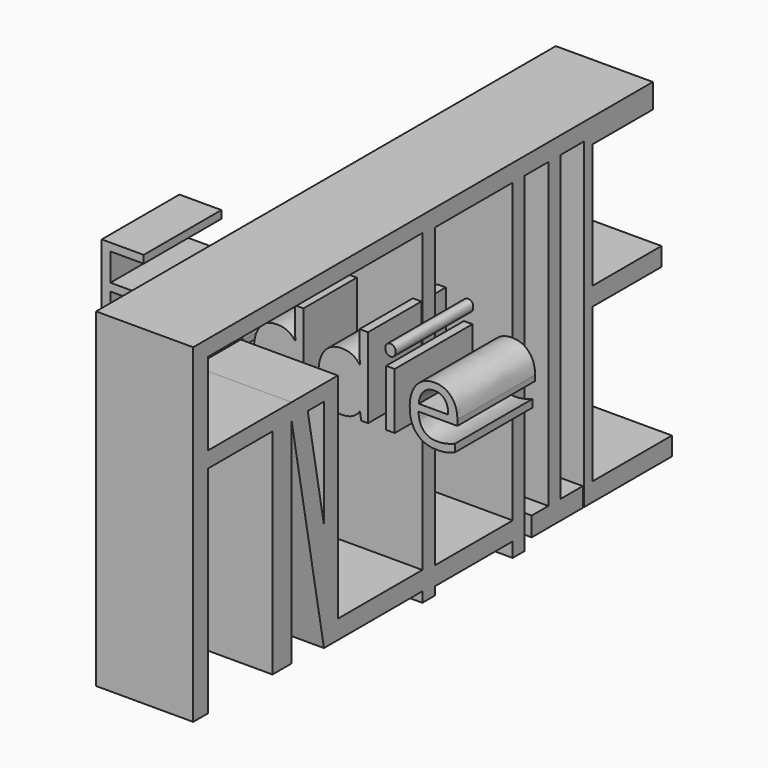
from build123d import *

# Parameters (mm, degrees)
F0_TEXT_SIZE = 27.5686564338
F1_DEPTH     = 25.4
F2_W         = 21.0011973977
F2_H         = 4.1624009609
F2_W_2       = 6.2435939908
F2_H_2       = 56.003193371
F2_W_3       = 27.6231979951
F2_H_3       = 4.9192011356
F2_W_4       = 4.0206052363
F2_H_4       = 79.2058780789
F2_H_5       = 5.025755614
F2_W_5       = 5.4278131574
F2_W_6       = 7.2370879352
F2_W_7       = 22.515386343
F2_H_6       = 4.8247235827
F2_W_8       = 25.9328857064
F2_H_7       = 4.8247240484
F3_DEPTH     = 25.4


# Not quite as in the source:
# - Text() gives the source's letters only with a copy of the font that has no kerning and outlines rounded to 1/6400 em; it was checked with that copy


with BuildPart() as f1:
    # F0 (on Front) → F1 (new body)
    with BuildSketch(Plane.XZ):
        with BuildLine():
            add(Edge.make_bspline(
                [(15.5439399558, 3.0433212141), (16.5799183734, 1.6024281552), (18.58726117, 1.6024281552)],
                knots=[0, 0, 0, 1, 1, 1], degree=2))
            add(Edge.make_bspline(
                [(18.58726117, 1.6024281552), (20.8745981335, 1.6024281552), (21.9041151472, 2.8473252973)],
                knots=[0, 0, 0, 1, 1, 1], degree=2))
            add(Edge.make_bspline(
                [(21.9041151472, 2.8473252973), (22.9336321609, 4.0922224394), (22.9336321609, 6.866318493)],
                knots=[0, 0, 0, 1, 1, 1], degree=2))
            Line((22.9336321609, 6.866318493), (22.9336321609, 7.3358471729))
            add(Edge.make_bspline(
                [(22.9336321609, 7.3358471729), (22.9336321609, 10.4717818423), (21.8911923395, 11.8114462409)],
                knots=[0, 0, 0, 1, 1, 1], degree=2))
            add(Edge.make_bspline(
                [(21.8911923395, 11.8114462409), (20.8487525181, 13.1511106394), (18.5614155546, 13.1511106394)],
                knots=[0, 0, 0, 1, 1, 1], degree=2))
            add(Edge.make_bspline(
                [(18.5614155546, 13.1511106394), (16.5928411811, 13.1511106394), (15.5504013597, 11.6240655292)],
                knots=[0, 0, 0, 1, 1, 1], degree=2))
            add(Edge.make_bspline(
                [(15.5504013597, 11.6240655292), (14.5079615383, 10.0970204189), (14.5079615383, 7.3100015575)],
                knots=[0, 0, 0, 1, 1, 1], degree=2))
            add(Edge.make_bspline(
                [(14.5079615383, 7.3100015575), (14.5079615383, 4.4842142731), (15.5439399558, 3.0433212141)],
                knots=[0, 0, 0, 1, 1, 1], degree=2))
        make_face()
        with BuildLine():
            add(Edge.make_bspline(
                [(-1.350477315, 3.0433212141), (-0.3144988974, 1.6024281552), (1.6928438991, 1.6024281552)],
                knots=[0, 0, 0, 1, 1, 1], degree=2))
            add(Edge.make_bspline(
                [(1.6928438991, 1.6024281552), (3.9801808626, 1.6024281552), (5.0096978763, 2.8473252973)],
                knots=[0, 0, 0, 1, 1, 1], degree=2))
            add(Edge.make_bspline(
                [(5.0096978763, 2.8473252973), (6.03921489, 4.0922224394), (6.03921489, 6.866318493)],
                knots=[0, 0, 0, 1, 1, 1], degree=2))
            Line((6.03921489, 6.866318493), (6.03921489, 7.3358471729))
            add(Edge.make_bspline(
                [(6.03921489, 7.3358471729), (6.03921489, 10.4717818423), (4.9967750686, 11.8114462409)],
                knots=[0, 0, 0, 1, 1, 1], degree=2))
            add(Edge.make_bspline(
                [(4.9967750686, 11.8114462409), (3.9543352472, 13.1511106394), (1.6669982837, 13.1511106394)],
                knots=[0, 0, 0, 1, 1, 1], degree=2))
            add(Edge.make_bspline(
                [(1.6669982837, 13.1511106394), (-0.3015760897, 13.1511106394), (-1.3440159111, 11.6240655292)],
                knots=[0, 0, 0, 1, 1, 1], degree=2))
            add(Edge.make_bspline(
                [(-1.3440159111, 11.6240655292), (-2.3864557326, 10.0970204189), (-2.3864557326, 7.3100015575)],
                knots=[0, 0, 0, 1, 1, 1], degree=2))
            add(Edge.make_bspline(
                [(-2.3864557326, 7.3100015575), (-2.3864557326, 4.4842142731), (-1.350477315, 3.0433212141)],
                knots=[0, 0, 0, 1, 1, 1], degree=2))
        make_face()
        with BuildLine():
            add(Edge.make_bspline(
                [(-11.0296602848, 12.0268263692), (-11.9708714459, 13.1511106394), (-13.7240656909, 13.1511106394)],
                knots=[0, 0, 0, 1, 1, 1], degree=2))
            add(Edge.make_bspline(
                [(-13.7240656909, 13.1511106394), (-15.4987979489, 13.1511106394), (-16.5563143793, 11.99451935)],
                knots=[0, 0, 0, 1, 1, 1], degree=2))
            add(Edge.make_bspline(
                [(-16.5563143793, 11.99451935), (-17.6138308097, 10.8379280605), (-17.8033653226, 8.7918168408)],
                knots=[0, 0, 0, 1, 1, 1], degree=2))
            Line((-17.8033653226, 8.7918168408), (-10.0884491237, 8.7918168408))
            add(Edge.make_bspline(
                [(-10.0884491237, 8.7918168408), (-10.0884491237, 10.902542099), (-11.0296602848, 12.0268263692)],
                knots=[0, 0, 0, 1, 1, 1], degree=2))
        make_face()
        with Locations((-47.2027528477, 0)):
            Text('Freddie', F0_TEXT_SIZE, font='Open Sans', text_align=(TextAlign.LEFT, TextAlign.BOTTOM))
    extrude(amount=F1_DEPTH)


with BuildPart() as f3:
    # F2 (on Right) → F3 (new body)
    with BuildSketch(Plane.YZ):
        Polygon((-77.9526382685, 40.9287288785), (-82.8718394041, 40.9287288785), (-82.8718394041, -45.3464612365), (-77.9526382685, -45.3464612365), (-77.9526382685, 11.0351322219), (-77.9526382685, 15.1975331828), (-77.9526382685, 36.7663279176), align=None)
        Polygon((-35.9502434731, 40.9287288785), (-77.9526382685, 40.9287288785), (-77.9526382685, 36.7663279176), (-56.9514408708, 36.7663279176), (-50.70784688, 36.7663279176), (-40.112644434, 36.7663279176), (-35.9502434731, 36.7663279176), align=None)
        Polygon((-7.9486491159, 40.9287288785), (-35.9502434731, 40.9287288785), (-35.9502434731, 36.7663279176), (-35.571847111, 36.7663279176), (-7.9486491159, 36.7663279176), align=None)
        with Locations((-67.4520395696, 13.1163327023)):
            Rectangle(F2_W, F2_H)
        Polygon((-3.7862497848, 40.9287288785), (-7.9486491159, 40.9287288785), (-7.9486491159, 36.7663279176), (-7.9486491159, 15.1975331828), (-7.9486491159, 11.0351322219), (-7.9486491159, -40.8056601882), (-7.9486491159, -45.7248613238), (-7.9486491159, -48.37365821), (-3.7862497848, -48.37365821), (-3.7862497848, -46.236936003), (-3.7862497848, -41.4122119546), (-3.7862497848, 36.3864563406), align=None)
        with Locations((-53.8296438754, 13.1163327023)):
            Rectangle(F2_W_2, F2_H)
        Polygon((25.4113916308, 40.9287288785), (-3.7862497848, 40.9287288785), (-3.7862497848, 36.3864563406), (6.916618906, 36.3864563406), (10.7361916453, 36.3864563406), (21.5918216854, 36.3864563406), (25.4113916308, 36.3864563406), align=None)
        with Locations((-53.8296438754, -16.9664644636)):
            Rectangle(F2_W_2, F2_H_2)
        Polygon((-40.112644434, 15.1975331828), (-50.70784688, 15.1975331828), (-50.70784688, 11.0351322219), (-45.410245657, 11.0351322219), (-40.112644434, 11.0351322219), (-35.571847111, 11.0351322219), (-35.571847111, 15.1975331828), align=None)
        Polygon((44.9113175273, 40.9287288785), (25.4113916308, 40.9287288785), (25.4113916308, 36.3864563406), (33.251568675, 36.3864563406), (37.2721739113, 36.3864563406), (44.9113175273, 36.3864563406), align=None)
        Polygon((-45.410245657, 11.0351322219), (-50.70784688, 11.0351322219), (-40.112644434, -45.7248613238), (-40.112644434, -17.344864551), align=None)
        Polygon((-35.571847111, -40.8056601882), (-35.571847111, 11.0351322219), (-40.112644434, 11.0351322219), (-40.112644434, 6.4943348989), (-40.112644434, -17.344864551), (-40.112644434, -45.7248613238), (-35.571847111, -45.7248613238), align=None)
        Polygon((6.916618906, -41.4122119546), (-3.7862497848, -41.4122119546), (-3.7862497848, -46.236936003), (21.5918216854, -46.236936003), (21.5918216854, -41.4122119546), (10.7361916453, -41.4122119546), align=None)
        Polygon((25.4113916308, -50.0565059483), (25.4113916308, 36.3864563406), (21.5918216854, 36.3864563406), (21.5918216854, -41.4122119546), (21.5918216854, -46.236936003), (21.5918216854, -50.0565059483), align=None)
        Polygon((67.4266889691, 40.9287288785), (44.9113175273, 40.9287288785), (44.9113175273, 36.3864563406), (44.9113175273, 34.5771871507), (47.7257370949, 34.5771871507), (67.4266889691, 34.5771871507), align=None)
        with Locations((-21.7602481134, -43.265260756)):
            Rectangle(F2_W_3, F2_H_3)
        with Locations((35.2618712932, -3.2164826989)):
            Rectangle(F2_W_4, F2_H_4)
        with Locations((35.2618712932, -45.3322995454)):
            Rectangle(F2_W_4, F2_H_5)
        with Locations((30.5376620963, -45.3322995454)):
            Rectangle(F2_W_5, F2_H_5)
        Polygon((47.7257370949, 34.5771871507), (44.9113175273, 34.5771871507), (44.9113175273, -47.8451773524), (47.7257370949, -47.8451773524), (47.7257370949, -43.0204533041), (47.7257370949, -2.8144221287), (47.7257370949, 2.010301454), align=None)
        with Locations((40.8907178789, -45.3322995454)):
            Rectangle(F2_W_6, F2_H_5)
        with Locations((58.9834302664, -0.4020603374)):
            Rectangle(F2_W_7, F2_H_6)
        with Locations((60.6921799481, -45.4328153282)):
            Rectangle(F2_W_8, F2_H_7)
    extrude(amount=F3_DEPTH)


solid = Compound([f1.part, f3.part])
